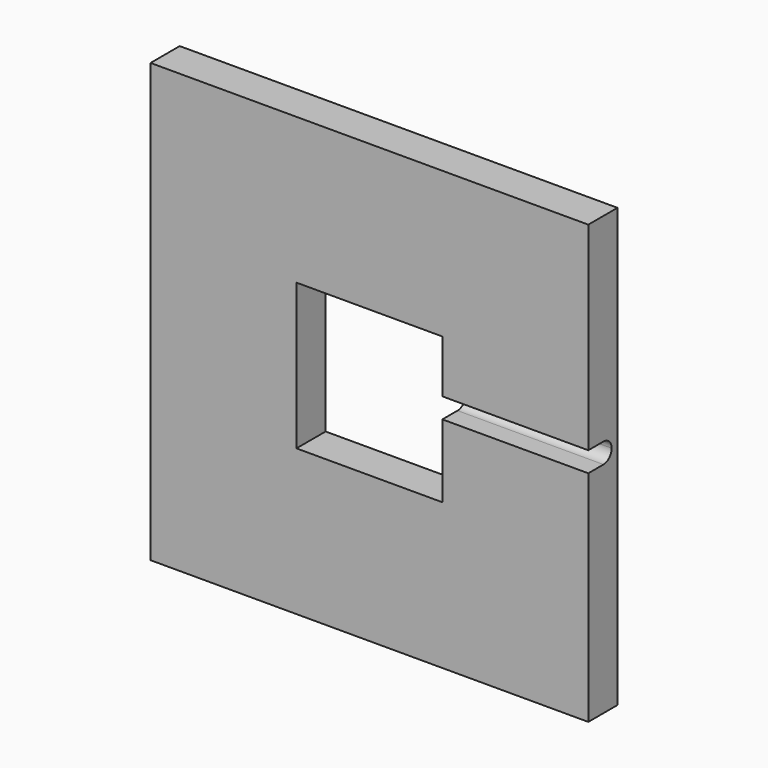
from build123d import *

# Parameters (mm, degrees)
F0_W        = 76.2
F0_H        = 6.35
F1_DEPTH    = 76.2
F2_W        = 25.4
F2_H        = 25.4
F3_DEPTH    = 25.4
F4_W        = 25.4
F4_H        = 3.5260361671
F5_DEPTH    = 5.08
F8_T1_DEPTH = 25.4


# Not quite as in the source:
# - a fillet or chamfer that OpenCascade refuses, or shapes differently, is made with other operations: its cross-section is extruded or revolved along the edge and cut away or added
# - the program builds the solid bodies; features that only make, move or delete a surface that nothing else refers to are left out


with BuildPart() as f1:
    # F0 (on Top) → F1 (new body)
    with BuildSketch(Plane.XY):
        Rectangle(F0_W, F0_H)
    extrude(amount=F1_DEPTH)

    # F2 (on face) → F3 (cut)
    with BuildSketch(Plane.XZ.offset(3.175)):
        with Locations((0, 38.1)):
            Rectangle(F2_W, F2_H)
    extrude(amount=-F3_DEPTH, mode=Mode.SUBTRACT)

    # F4 (on face) → F5 (cut)
    with BuildSketch(Plane.XZ.offset(3.175)):
        with Locations((25.4, 39.8630180836)):
            Rectangle(F4_W, F4_H)
    extrude(amount=-F5_DEPTH, mode=Mode.SUBTRACT)

    # F8: fillet of radius 1.778 on 2 edges, made by hand

    # F8_s2 → F8_t1 (join)
    with BuildSketch(Plane.YZ.offset(12.7)):
        with BuildLine():
            ThreePointArc((0.127, 41.6260361671), (1.3842358569, 41.1052720241), (1.905, 39.8480361671))
            Line((1.905, 39.8480361671), (1.905, 41.6260361671))
            Line((1.905, 41.6260361671), (0.127, 41.6260361671))
        make_face()
        with BuildLine():
            ThreePointArc((0.127, 38.1), (1.3842358569, 38.6207641431), (1.905, 39.878))
            Line((1.905, 39.878), (1.905, 38.1))
            Line((1.905, 38.1), (0.127, 38.1))
        make_face()
    extrude(amount=F8_T1_DEPTH)


solid = f1.part
